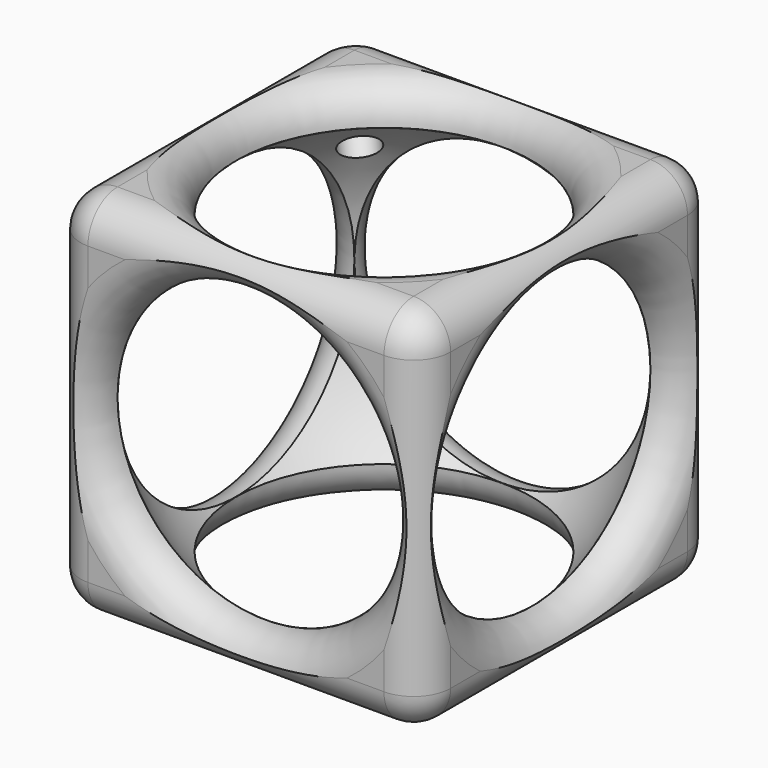
from build123d import *

# Parameters (mm, degrees)
F0_W         = 50
F0_H         = 50
F1_DEPTH     = 50
F4_R         = 20
F5_DEPTH     = 50
F3_R         = 20
F6_DEPTH     = 50
F2_R         = 20
F7_DEPTH     = 50
F8_F1_R      = 4.9999
F8_F2_R      = 4.9999
F8_F3_R      = 4.9999
F8_F4_R      = 4.9999
F8_F5_R      = 4.9999
F8_F6_R      = 4.9999
F8_T7_DEPTH  = 75
F8_T9_DEPTH  = 57.5
F8_T11_DEPTH = 57.5
F8_T14_ANGLE = 90
F8_T15_DEPTH = 57.5
F8_T17_DEPTH = 57.5
F8_T20_ANGLE = 90
F8_T21_DEPTH = 40
F8_T23_DEPTH = 57.5
F8_T26_ANGLE = 90
F8_T28_ANGLE = 90
F8_T29_DEPTH = 40
F8_T31_DEPTH = 40
F8_T34_ANGLE = 90
F8_T36_ANGLE = 90
F8_T38_ANGLE = 90
F8_T40_ANGLE = 90
F12_R        = 2.5
F13_DEPTH    = 50
F14_R        = 0.5


# Not quite as in the source:
# - a fillet or chamfer that OpenCascade refuses, or shapes differently, is made with other operations: its cross-section is extruded or revolved along the edge and cut away or added
# - a fillet or chamfer is up to 0.001 mm smaller than in the source, because OpenCascade refuses the exact size


with BuildPart() as f1:
    # F0 (on Top) → F1 (new body)
    with BuildSketch(Plane.XY):
        Rectangle(F0_W, F0_H)
    extrude(amount=F1_DEPTH)

    # F4 (on face) → F5 (cut)
    with BuildSketch(Plane.XY.offset(50)):
        Circle(F4_R)
    extrude(amount=-F5_DEPTH, mode=Mode.SUBTRACT)

    # F3 (on face) → F6 (cut)
    with BuildSketch(Plane(origin=(0, 25, 0), x_dir=(-1, 0, 0), z_dir=(0, 1, 0))):
        with Locations((0, 25)):
            Circle(F3_R)
    extrude(amount=-F6_DEPTH, mode=Mode.SUBTRACT)

    # F2 (on face) → F7 (cut)
    with BuildSketch(Plane(origin=(-25, 0, 0), x_dir=(0, -1, 0), z_dir=(-1, 0, 0))):
        with Locations((0, 25)):
            Circle(F2_R)
    extrude(amount=-F7_DEPTH, mode=Mode.SUBTRACT)

    # F8: fillet of radius 5 on 18 edges, made by hand

    # F8_f1 (radius 5 in the source; OpenCascade refuses exactly that, so slightly less here)
    f8_f1_edges = [f1.edges().sort_by_distance(p)[0] for p in [
        (-25, 20, 25),
    ]]
    fillet(f8_f1_edges, radius=F8_F1_R)

    # F8_f2 (radius 5 in the source; OpenCascade refuses exactly that, so slightly less here)
    f8_f2_edges = [f1.edges().sort_by_distance(p)[0] for p in [
        (20, 25, 25),
    ]]
    fillet(f8_f2_edges, radius=F8_F2_R)

    # F8_f3 (radius 5 in the source; OpenCascade refuses exactly that, so slightly less here)
    f8_f3_edges = [f1.edges().sort_by_distance(p)[0] for p in [
        (-20, 0, 0),
    ]]
    fillet(f8_f3_edges, radius=F8_F3_R)

    # F8_f4 (radius 5 in the source; OpenCascade refuses exactly that, so slightly less here)
    f8_f4_edges = [f1.edges().sort_by_distance(p)[0] for p in [
        (-20, 0, 50),
    ]]
    fillet(f8_f4_edges, radius=F8_F4_R)

    # F8_f5 (radius 5 in the source; OpenCascade refuses exactly that, so slightly less here)
    f8_f5_edges = [f1.edges().sort_by_distance(p)[0] for p in [
        (20, -25, 25),
    ]]
    fillet(f8_f5_edges, radius=F8_F5_R)

    # F8_f6 (radius 5 in the source; OpenCascade refuses exactly that, so slightly less here)
    f8_f6_edges = [f1.edges().sort_by_distance(p)[0] for p in [
        (25, 20, 25),
    ]]
    fillet(f8_f6_edges, radius=F8_F6_R)

    # F8_s8 → F8_t7 (cut)
    with BuildSketch(Plane.XY.offset(-12.5)):
        with BuildLine():
            ThreePointArc((-20, 25), (-23.5355339059, 23.5355339059), (-25, 20))
            Line((-25, 20), (-25.1, 20))
            Line((-25.1, 20), (-25.1, 25.1))
            Line((-25.1, 25.1), (-20, 25.1))
            Line((-20, 25.1), (-20, 25))
        make_face()
    extrude(amount=F8_T7_DEPTH, mode=Mode.SUBTRACT)

    # F8_s10 → F8_t9 (cut)
    with BuildSketch(Plane.XZ.offset(-20)):
        with BuildLine():
            ThreePointArc((-20, 0), (-23.5355339059, 1.4644660941), (-25, 5))
            Line((-25, 5), (-25.1, 5))
            Line((-25.1, 5), (-25.1, -0.1))
            Line((-25.1, -0.1), (-20, -0.1))
            Line((-20, -0.1), (-20, 0))
        make_face()
    extrude(amount=F8_T9_DEPTH, mode=Mode.SUBTRACT)

    # F8_s12 → F8_t11 (cut)
    with BuildSketch(Plane.YZ.offset(-20)):
        with BuildLine():
            ThreePointArc((20, 0), (23.5355339059, 1.4644660941), (25, 5))
            Line((25, 5), (25.1, 5))
            Line((25.1, 5), (25.1, -0.1))
            Line((25.1, -0.1), (20, -0.1))
            Line((20, -0.1), (20, 0))
        make_face()
    extrude(amount=F8_T11_DEPTH, mode=Mode.SUBTRACT)

    # F8_s13 → F8_t14 (revolve, cut)
    with BuildSketch(Plane.XZ.offset(-20)):
        with BuildLine():
            ThreePointArc((-20, 0), (-23.5355339059, 1.4644660941), (-25, 5))
            Line((-25, 5), (-25.1, 5))
            Line((-25.1, 5), (-25.1, -0.1))
            Line((-25.1, -0.1), (-20, -0.1))
            Line((-20, -0.1), (-20, 0))
        make_face()
    revolve(axis=Axis((-20, 20, 0), (0, 0, -1)), revolution_arc=F8_T14_ANGLE, mode=Mode.SUBTRACT)

    # F8_s16 → F8_t15 (cut)
    with BuildSketch(Plane.XZ.offset(-20)):
        with BuildLine():
            ThreePointArc((-20, 50), (-23.5355339059, 48.5355339059), (-25, 45))
            Line((-25, 45), (-25.1, 45))
            Line((-25.1, 45), (-25.1, 50.1))
            Line((-25.1, 50.1), (-20, 50.1))
            Line((-20, 50.1), (-20, 50))
        make_face()
    extrude(amount=F8_T15_DEPTH, mode=Mode.SUBTRACT)

    # F8_s18 → F8_t17 (cut)
    with BuildSketch(Plane.YZ.offset(-20)):
        with BuildLine():
            ThreePointArc((25, 45), (23.5355339059, 48.5355339059), (20, 50))
            Line((20, 50), (20, 50.1))
            Line((20, 50.1), (25.1, 50.1))
            Line((25.1, 50.1), (25.1, 45))
            Line((25.1, 45), (25, 45))
        make_face()
    extrude(amount=F8_T17_DEPTH, mode=Mode.SUBTRACT)

    # F8_s19 → F8_t20 (revolve, cut)
    with BuildSketch(Plane.XZ.offset(-20)):
        with BuildLine():
            ThreePointArc((-20, 50), (-23.5355339059, 48.5355339059), (-25, 45))
            Line((-25, 45), (-25.1, 45))
            Line((-25.1, 45), (-25.1, 50.1))
            Line((-25.1, 50.1), (-20, 50.1))
            Line((-20, 50.1), (-20, 50))
        make_face()
    revolve(axis=Axis((-20, 20, 50), (0, 0, -1)), revolution_arc=F8_T20_ANGLE, mode=Mode.SUBTRACT)

    # F8_s22 → F8_t21 (cut)
    with BuildSketch(Plane.XY.offset(5)):
        with BuildLine():
            ThreePointArc((-20, -25), (-23.5355339059, -23.5355339059), (-25, -20))
            Line((-25, -20), (-25.1, -20))
            Line((-25.1, -20), (-25.1, -25.1))
            Line((-25.1, -25.1), (-20, -25.1))
            Line((-20, -25.1), (-20, -25))
        make_face()
    extrude(amount=F8_T21_DEPTH, mode=Mode.SUBTRACT)

    # F8_s24 → F8_t23 (cut)
    with BuildSketch(Plane.YZ.offset(-20)):
        with BuildLine():
            ThreePointArc((-20, 50), (-23.5355339059, 48.5355339059), (-25, 45))
            Line((-25, 45), (-25.1, 45))
            Line((-25.1, 45), (-25.1, 50.1))
            Line((-25.1, 50.1), (-20, 50.1))
            Line((-20, 50.1), (-20, 50))
        make_face()
        with BuildLine():
            ThreePointArc((-20, 0), (-23.5355339059, 1.4644660941), (-25, 5))
            Line((-25, 5), (-25.1, 5))
            Line((-25.1, 5), (-25.1, -0.1))
            Line((-25.1, -0.1), (-20, -0.1))
            Line((-20, -0.1), (-20, 0))
        make_face()
    extrude(amount=F8_T23_DEPTH, mode=Mode.SUBTRACT)

    # F8_s25 → F8_t26 (revolve, cut)
    with BuildSketch(Plane.YZ.offset(-20)):
        with BuildLine():
            ThreePointArc((-25, 5), (-23.5355339059, 1.4644660941), (-20, 0))
            Line((-20, 0), (-20, -0.1))
            Line((-20, -0.1), (-25.1, -0.1))
            Line((-25.1, -0.1), (-25.1, 5))
            Line((-25.1, 5), (-25, 5))
        make_face()
    revolve(axis=Axis((-20, -25, 5), (0, 1, 0)), revolution_arc=F8_T26_ANGLE, mode=Mode.SUBTRACT)

    # F8_s27 → F8_t28 (revolve, cut)
    with BuildSketch(Plane.XY.offset(45)):
        with BuildLine():
            ThreePointArc((-20, -25), (-23.5355339059, -23.5355339059), (-25, -20))
            Line((-25, -20), (-25.1, -20))
            Line((-25.1, -20), (-25.1, -25.1))
            Line((-25.1, -25.1), (-20, -25.1))
            Line((-20, -25.1), (-20, -25))
        make_face()
    revolve(axis=Axis((-20, -25, 45), (0, 1, 0)), revolution_arc=F8_T28_ANGLE, mode=Mode.SUBTRACT)

    # F8_s30 → F8_t29 (cut)
    with BuildSketch(Plane.XY.offset(5)):
        with BuildLine():
            ThreePointArc((25, 20), (23.5355339059, 23.5355339059), (20, 25))
            Line((20, 25), (20, 25.1))
            Line((20, 25.1), (25.1, 25.1))
            Line((25.1, 25.1), (25.1, 20))
            Line((25.1, 20), (25, 20))
        make_face()
        with BuildLine():
            ThreePointArc((25, -20), (23.5355339059, -23.5355339059), (20, -25))
            Line((20, -25), (20, -25.1))
            Line((20, -25.1), (25.1, -25.1))
            Line((25.1, -25.1), (25.1, -20))
            Line((25.1, -20), (25, -20))
        make_face()
    extrude(amount=F8_T29_DEPTH, mode=Mode.SUBTRACT)

    # F8_s32 → F8_t31 (cut)
    with BuildSketch(Plane.XZ.offset(-20)):
        with BuildLine():
            ThreePointArc((25, 45), (23.5355339059, 48.5355339059), (20, 50))
            Line((20, 50), (20, 50.1))
            Line((20, 50.1), (25.1, 50.1))
            Line((25.1, 50.1), (25.1, 45))
            Line((25.1, 45), (25, 45))
        make_face()
        with BuildLine():
            ThreePointArc((25, 5), (23.5355339059, 1.4644660941), (20, 0))
            Line((20, 0), (20, -0.1))
            Line((20, -0.1), (25.1, -0.1))
            Line((25.1, -0.1), (25.1, 5))
            Line((25.1, 5), (25, 5))
        make_face()
    extrude(amount=F8_T31_DEPTH, mode=Mode.SUBTRACT)

    # F8_s33 → F8_t34 (revolve, cut)
    with BuildSketch(Plane.XZ.offset(-20)):
        with BuildLine():
            ThreePointArc((25, 5), (23.5355339059, 1.4644660941), (20, 0))
            Line((20, 0), (20, -0.1))
            Line((20, -0.1), (25.1, -0.1))
            Line((25.1, -0.1), (25.1, 5))
            Line((25.1, 5), (25, 5))
        make_face()
    revolve(axis=Axis((25, 20, 5), (1, 0, 0)), revolution_arc=F8_T34_ANGLE, mode=Mode.SUBTRACT)

    # F8_s35 → F8_t36 (revolve, cut)
    with BuildSketch(Plane.XY.offset(45)):
        with BuildLine():
            ThreePointArc((25, 20), (23.5355339059, 23.5355339059), (20, 25))
            Line((20, 25), (20, 25.1))
            Line((20, 25.1), (25.1, 25.1))
            Line((25.1, 25.1), (25.1, 20))
            Line((25.1, 20), (25, 20))
        make_face()
    revolve(axis=Axis((25, 20, 45), (1, 0, 0)), revolution_arc=F8_T36_ANGLE, mode=Mode.SUBTRACT)

    # F8_s37 → F8_t38 (revolve, cut)
    with BuildSketch(Plane.XY.offset(45)):
        with BuildLine():
            ThreePointArc((25, -20), (23.5355339059, -23.5355339059), (20, -25))
            Line((20, -25), (20, -25.1))
            Line((20, -25.1), (25.1, -25.1))
            Line((25.1, -25.1), (25.1, -20))
            Line((25.1, -20), (25, -20))
        make_face()
    revolve(axis=Axis((25, -20, 45), (-1, 0, 0)), revolution_arc=F8_T38_ANGLE, mode=Mode.SUBTRACT)

    # F8_s39 → F8_t40 (revolve, cut)
    with BuildSketch(Plane.XZ.offset(20)):
        with BuildLine():
            ThreePointArc((25, 5), (23.5355339059, 1.4644660941), (20, 0))
            Line((20, 0), (20, -0.1))
            Line((20, -0.1), (25.1, -0.1))
            Line((25.1, -0.1), (25.1, 5))
            Line((25.1, 5), (25, 5))
        make_face()
    revolve(axis=Axis((25, -20, 5), (-1, 0, 0)), revolution_arc=F8_T40_ANGLE, mode=Mode.SUBTRACT)

    # F9 (on Front) → F10 (revolve, cut)
    with BuildSketch(Plane.XZ):
        with BuildLine():
            Line((0, 25), (0, 0))
            Line((0, 0), (0, -3.275))
            ThreePointArc((0, -3.275), (19.993444238, 5.006555762), (28.275, 25))
            ThreePointArc((28.275, 25), (19.993444238, 44.993444238), (0, 53.275))
            Line((0, 53.275), (0, 25))
        make_face()
    revolve(axis=Axis((0, 0, 25), (0, 0, 1)), mode=Mode.SUBTRACT)

    # F12 (on face) → F13 (cut, symmetric)
    with BuildSketch(Plane(origin=(-30, 30, 30), x_dir=(0.8164965809, 0.4082482905, 0.4082482905), z_dir=(0.5773502692, -0.5773502692, -0.5773502692))):
        with Locations((10.1675949991, 17.6499933004)):
            Circle(F12_R)
    extrude(amount=F13_DEPTH, both=True, mode=Mode.SUBTRACT)

    # F14
    f14_edges = [f1.edges().sort_by_distance(p)[0] for p in [
        (-24.559223, 21.423, 46.479376),
    ]]
    fillet(f14_edges, radius=F14_R)


solid = f1.part
